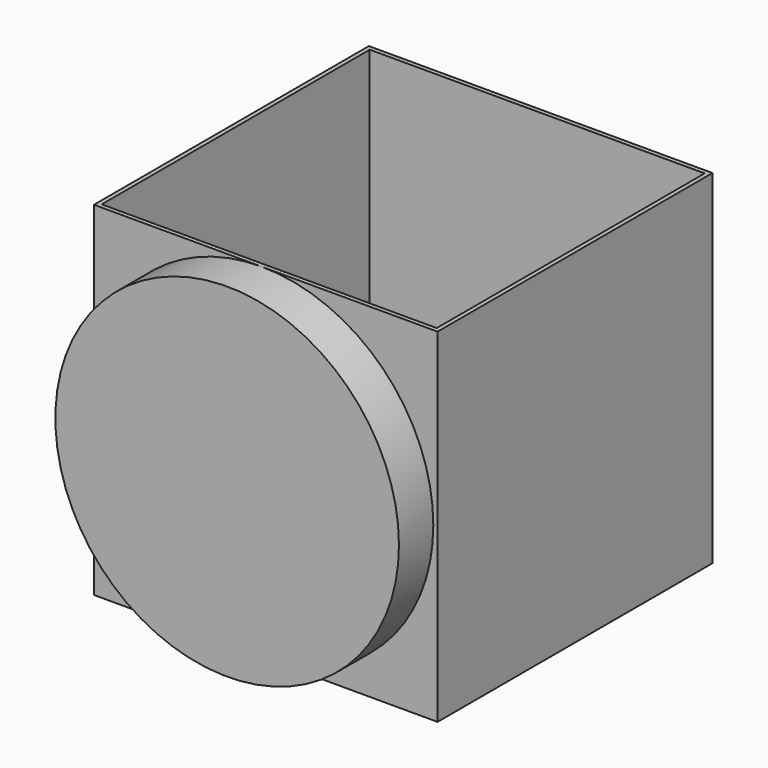
from build123d import *

# Parameters (mm, degrees)
F0_W     = 200
F0_H     = 200
F1_DEPTH = 200
F4_T     = -2.5
F5_R     = 100
F6_DEPTH = 25


# Not quite as in the source:
# - the program builds the solid bodies; features that only make, move or delete a surface that nothing else refers to are left out


with BuildPart() as f1:
    # F0 (on Front) → F1 (new body)
    with BuildSketch(Plane.XZ):
        with Locations((2.4823185522, 0)):
            Rectangle(F0_W, F0_H)
    extrude(amount=-F1_DEPTH)

    # F4
    f4_openings = [f1.faces().sort_by_distance(p)[0] for p in [
        (2.482319, 100, 100),
    ]]
    offset(amount=F4_T, openings=f4_openings)

    # F5 (on face) → F6 (join)
    with BuildSketch(Plane.XZ):
        Circle(F5_R)
    extrude(amount=F6_DEPTH)


solid = f1.part
